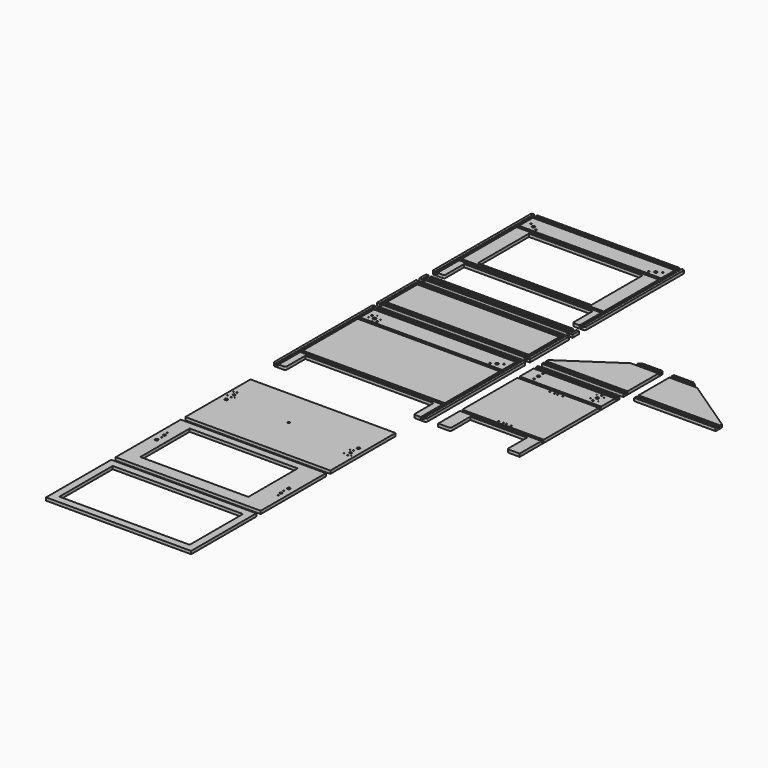
from build123d import *

# Parameters (mm, degrees)
F0_W     = 576
F0_H     = 12
F0_W_2   = 10
F0_H_2   = 505
F0_H_3   = 70
F0_W_3   = 460
F0_H_4   = 50
F0_H_5   = 10
F0_H_6   = 279
F0_H_7   = 259
F0_W_4   = 6
F1_DEPTH = 12
F0_W_5   = 330
F0_W_6   = 588
F0_H_8   = 330
F0_R     = 4.7874665738
F0_W_7   = 438
F0_H_9   = 250
F0_W_8   = 528
F0_H_10  = 270
F0_H_11  = 156
F0_W_9   = 12
F2_DEPTH = 6
F3_R     = 6
F3_R_2   = 2.5
F3_R_3   = 3.3
F3_R_4   = 5
F4_DEPTH = 25
F5_R     = 7
F5_2_R   = 7
F5_3_R   = 7
F6_R     = 1.5
F7_DEPTH = 25


with BuildPart() as f1:
    # F0 (on Top) → F1 (new body)
    with BuildSketch(Plane.XY):
        with Locations((151.8414666056, 1212)):
            Rectangle(F0_W, F0_H)
        with Locations((456.8414666056, 1057.5)):
            Rectangle(F0_W_2, F0_H_2)
        with Locations((151.8414666056, 921)):
            Rectangle(F0_W, F0_H)
        with Locations((151.8414666056, 1253)):
            Rectangle(F0_W, F0_H_3)
        with Locations((151.8414666056, 1253)):
            Rectangle(F0_W_3, F0_H_4, mode=Mode.SUBTRACT)
        with Locations((151.8414666056, 1305)):
            Rectangle(F0_W, F0_H_5)
        with Locations((151.8414666056, 1294)):
            Rectangle(F0_W, F0_H)
        with Locations((151.8414666056, 1066.5)):
            Rectangle(F0_W, F0_H_6)
        with Locations((151.8414666056, 1066.5)):
            Rectangle(F0_W_3, F0_H_7, mode=Mode.SUBTRACT)
        Polygon((-136.1585333944, 915), (-136.1585333944, 805), (-108.1585333944, 805), (-108.1585333944, 905), (411.8414666056, 905), (411.8414666056, 805), (439.8414666056, 805), (439.8414666056, 915), align=None)
        with Locations((-153.1585333944, 1057.5)):
            Rectangle(F0_W_2, F0_H_2)
        Polygon((-148.1585333944, 1310), (-148.1585333944, 805), (-136.1585333944, 805), (-136.1585333944, 915), (-142.1585333944, 915), (-142.1585333944, 927), (-136.1585333944, 927), (-136.1585333944, 1206), (-142.1585333944, 1206), (-142.1585333944, 1218), (-136.1585333944, 1218), (-136.1585333944, 1288), (-142.1585333944, 1288), (-142.1585333944, 1300), (-136.1585333944, 1300), (-136.1585333944, 1310), align=None)
        Polygon((451.8414666056, 1310), (439.8414666056, 1310), (439.8414666056, 1300), (445.8414666056, 1300), (445.8414666056, 1288), (439.8414666056, 1288), (439.8414666056, 1218), (445.8414666056, 1218), (445.8414666056, 1206), (439.8414666056, 1206), (439.8414666056, 927), (445.8414666056, 927), (445.8414666056, 915), (439.8414666056, 915), (439.8414666056, 805), (451.8414666056, 805), align=None)
        with Locations((442.8414666056, 921)):
            Rectangle(F0_W_4, F0_H)
        with Locations((-139.1585333944, 1212)):
            Rectangle(F0_W_4, F0_H)
        with Locations((442.8414666056, 1294)):
            Rectangle(F0_W_4, F0_H)
        with Locations((442.8414666056, 1212)):
            Rectangle(F0_W_4, F0_H)
        with Locations((-139.1585333944, 1294)):
            Rectangle(F0_W_4, F0_H)
        with Locations((-139.1585333944, 921)):
            Rectangle(F0_W_4, F0_H)
        with Locations((151.8414666056, 1253)):
            Rectangle(F0_W_3, F0_H_4)
    extrude(amount=-F1_DEPTH)


with BuildPart() as f1b:
    # F0 (on Top) → F1, piece 2 (new body)
    with BuildSketch(Plane.XY):
        with Locations((675.8917057514, 448)):
            Rectangle(F0_W_5, F0_H_3)
        with Locations((675.8917057514, 261.5)):
            Rectangle(F0_W_5, F0_H_6)
        with Locations((675.8917057514, 407)):
            Rectangle(F0_W_5, F0_H)
        Polygon((510.8917057514, 110), (510.8917057514, 0), (560.8917057514, 0), (560.8917057514, 100), (790.8917057514, 100), (790.8917057514, 0), (840.8917057514, 0), (840.8917057514, 110), align=None)
        with Locations((675.8917057514, 116)):
            Rectangle(F0_W_5, F0_H)
        with Locations((675.8917057514, 500)):
            Rectangle(F0_W_5, F0_H_5)
        with Locations((675.8917057514, 489)):
            Rectangle(F0_W_5, F0_H)
    extrude(amount=-F1_DEPTH)


with BuildPart() as f1c:
    # F0 (on Top) → F1, piece 3 (new body)
    with BuildSketch(Plane.XY):
        with Locations((151.8414666056, 261.5)):
            Rectangle(F0_W, F0_H_6)
        with Locations((151.8414666056, 500)):
            Rectangle(F0_W, F0_H_5)
        Polygon((-136.1585333944, 110), (-136.1585333944, 0), (-108.1585333944, 0), (-108.1585333944, 100), (411.8414666056, 100), (411.8414666056, 0), (439.8414666056, 0), (439.8414666056, 110), align=None)
        with Locations((151.8414666056, 407)):
            Rectangle(F0_W, F0_H)
        with Locations((151.8414666056, 448)):
            Rectangle(F0_W, F0_H_3)
        with Locations((-153.1585333944, 252.5)):
            Rectangle(F0_W_2, F0_H_2)
        with Locations((151.8414666056, 489)):
            Rectangle(F0_W, F0_H)
        with Locations((151.8414666056, 116)):
            Rectangle(F0_W, F0_H)
        with Locations((-139.1585333944, 407)):
            Rectangle(F0_W_4, F0_H)
        with Locations((-139.1585333944, 116)):
            Rectangle(F0_W_4, F0_H)
        with Locations((-139.1585333944, 489)):
            Rectangle(F0_W_4, F0_H)
        with Locations((456.8414666056, 252.5)):
            Rectangle(F0_W_2, F0_H_2)
        with Locations((442.8414666056, 489)):
            Rectangle(F0_W_4, F0_H)
        with Locations((442.8414666056, 116)):
            Rectangle(F0_W_4, F0_H)
        with Locations((442.8414666056, 407)):
            Rectangle(F0_W_4, F0_H)
        Polygon((-148.1585333944, 505), (-148.1585333944, 0), (-136.1585333944, 0), (-136.1585333944, 110), (-142.1585333944, 110), (-142.1585333944, 122), (-136.1585333944, 122), (-136.1585333944, 401), (-142.1585333944, 401), (-142.1585333944, 413), (-136.1585333944, 413), (-136.1585333944, 483), (-142.1585333944, 483), (-142.1585333944, 495), (-136.1585333944, 495), (-136.1585333944, 505), align=None)
        Polygon((451.8414666056, 505), (439.8414666056, 505), (439.8414666056, 495), (445.8414666056, 495), (445.8414666056, 483), (439.8414666056, 483), (439.8414666056, 413), (445.8414666056, 413), (445.8414666056, 401), (439.8414666056, 401), (439.8414666056, 122), (445.8414666056, 122), (445.8414666056, 110), (439.8414666056, 110), (439.8414666056, 0), (451.8414666056, 0), align=None)
    extrude(amount=-F1_DEPTH)


with BuildPart() as f1d:
    # F0 (on Top) → F1, piece 4 (new body)
    with BuildSketch(Plane.XY):
        with Locations((151.8414666056, -300.2730111413)):
            Rectangle(F0_W_6, F0_H_8)
        with Locations((136.8414666056, -290.2730111413)):
            Circle(F0_R, mode=Mode.SUBTRACT)
    extrude(amount=-F1_DEPTH)


with BuildPart() as f1e:
    # F0 (on Top) → F1, piece 5 (new body)
    with BuildSketch(Plane.XY):
        with Locations((151.8414666056, -653.3492064476)):
            Rectangle(F0_W_6, F0_H_8)
        with Locations((136.8414666056, -643.3492064476)):
            Rectangle(F0_W_7, F0_H_9, mode=Mode.SUBTRACT)
    extrude(amount=-F1_DEPTH)


with BuildPart() as f1f:
    # F0 (on Top) → F1, piece 6 (new body)
    with BuildSketch(Plane.XY):
        with Locations((151.8414666056, -1005.8201861382)):
            Rectangle(F0_W_6, F0_H_8)
        with Locations((151.8414666056, -1005.8201861382)):
            Rectangle(F0_W_8, F0_H_10, mode=Mode.SUBTRACT)
    extrude(amount=-F1_DEPTH)


with BuildPart() as f1g:
    # F0 (on Top) → F1, piece 7 (new body)
    with BuildSketch(Plane.XY):
        Polygon((510.8917057514, 557), (510.8917057514, 547), (840.8917057514, 547), (840.8917057514, 703), (728.1536105133, 703), align=None)
        Polygon((728.1536105133, 703), (840.8917057514, 703), (840.8917057514, 715), (746.0107533705, 715), align=None)
        Polygon((746.0107533705, 715), (840.8917057514, 715), (840.8917057514, 725), (760.8917057514, 725), align=None)
        with Locations((675.8917057514, 530)):
            Rectangle(F0_W_5, F0_H_5)
        with Locations((675.8917057514, 541)):
            Rectangle(F0_W_5, F0_H)
    extrude(amount=-F1_DEPTH)


with BuildPart() as f1h:
    # F0 (on Top) → F1, piece 8 (new body)
    with BuildSketch(Plane.XY):
        Polygon((885.1829600334, 703), (885.1829600334, 547), (1215.1829600334, 547), (1215.1829600334, 557), (997.9210552715, 703), align=None)
        Polygon((885.1829600334, 725), (885.1829600334, 715), (980.0639124144, 715), (965.1829600334, 725), align=None)
        Polygon((885.1829600334, 715), (885.1829600334, 703), (997.9210552715, 703), (980.0639124144, 715), align=None)
        with Locations((1050.1829600334, 530)):
            Rectangle(F0_W_5, F0_H_5)
        with Locations((1050.1829600334, 541)):
            Rectangle(F0_W_5, F0_H)
    extrude(amount=-F1_DEPTH)


with BuildPart() as f1i:
    # F0 (on Top) → F1, piece 9 (new body)
    with BuildSketch(Plane.XY):
        with Locations((151.8414666056, 625)):
            Rectangle(F0_W, F0_H_11)
        with Locations((151.8414666056, 709)):
            Rectangle(F0_W, F0_H)
        with Locations((151.8414666056, 720)):
            Rectangle(F0_W, F0_H_5)
        with Locations((-142.1585333944, 720)):
            Rectangle(F0_W_9, F0_H_5)
        with Locations((-142.1585333944, 709)):
            Rectangle(F0_W_9, F0_H)
        with Locations((-142.1585333944, 625)):
            Rectangle(F0_W_9, F0_H_11)
        Polygon((-148.1585333944, 725), (-158.1585333944, 725), (-158.1585333944, 525), (-148.1585333944, 525), (-148.1585333944, 535), (-148.1585333944, 547), (-148.1585333944, 703), (-148.1585333944, 715), align=None)
        Polygon((461.8414666056, 725), (451.8414666056, 725), (451.8414666056, 715), (451.8414666056, 703), (451.8414666056, 547), (451.8414666056, 535), (451.8414666056, 525), (461.8414666056, 525), align=None)
        with Locations((445.8414666056, 720)):
            Rectangle(F0_W_9, F0_H_5)
        with Locations((445.8414666056, 709)):
            Rectangle(F0_W_9, F0_H)
        with Locations((445.8414666056, 625)):
            Rectangle(F0_W_9, F0_H_11)
        with Locations((151.8414666056, 530)):
            Rectangle(F0_W, F0_H_5)
        with Locations((151.8414666056, 541)):
            Rectangle(F0_W, F0_H)
        with Locations((445.8414666056, 541)):
            Rectangle(F0_W_9, F0_H)
        with Locations((445.8414666056, 530)):
            Rectangle(F0_W_9, F0_H_5)
        with Locations((-142.1585333944, 541)):
            Rectangle(F0_W_9, F0_H)
        with Locations((-142.1585333944, 530)):
            Rectangle(F0_W_9, F0_H_5)
    extrude(amount=-F1_DEPTH)


with BuildPart() as f1j:
    # F0 (on Top) → F1, piece 10 (new body)
    with BuildSketch(Plane.XY):
        with Locations((151.8414666056, 768.795539856)):
            Rectangle(F0_W, F0_H_5)
        with Locations((151.8414666056, 757.795539856)):
            Rectangle(F0_W, F0_H)
        with Locations((151.8414666056, 746.795539856)):
            Rectangle(F0_W, F0_H_5)
        with Locations((445.8414666056, 757.795539856)):
            Rectangle(F0_W_9, F0_H)
        Polygon((451.8414666056, 751.795539856), (451.8414666056, 741.795539856), (461.8414666056, 741.795539856), (461.8414666056, 773.795539856), (451.8414666056, 773.795539856), (451.8414666056, 763.795539856), align=None)
        with Locations((445.8414666056, 746.795539856)):
            Rectangle(F0_W_9, F0_H_5)
        with Locations((445.8414666056, 768.795539856)):
            Rectangle(F0_W_9, F0_H_5)
        Polygon((-158.1585333944, 773.795539856), (-158.1585333944, 741.795539856), (-148.1585333944, 741.795539856), (-148.1585333944, 751.795539856), (-148.1585333944, 763.795539856), (-148.1585333944, 773.795539856), align=None)
        with Locations((-142.1585333944, 757.795539856)):
            Rectangle(F0_W_9, F0_H)
        with Locations((-142.1585333944, 768.795539856)):
            Rectangle(F0_W_9, F0_H_5)
        with Locations((-142.1585333944, 746.795539856)):
            Rectangle(F0_W_9, F0_H_5)
    extrude(amount=-F1_DEPTH)


with BuildPart() as f2_tool:
    # F0 (on Top) → F2 (new body)
    with BuildSketch(Plane.XY):
        with Locations((151.8414666056, 1212)):
            Rectangle(F0_W, F0_H)
        with Locations((151.8414666056, 1294)):
            Rectangle(F0_W, F0_H)
        with Locations((151.8414666056, 921)):
            Rectangle(F0_W, F0_H)
        Polygon((-148.1585333944, 1310), (-148.1585333944, 805), (-136.1585333944, 805), (-136.1585333944, 915), (-142.1585333944, 915), (-142.1585333944, 927), (-136.1585333944, 927), (-136.1585333944, 1206), (-142.1585333944, 1206), (-142.1585333944, 1218), (-136.1585333944, 1218), (-136.1585333944, 1288), (-142.1585333944, 1288), (-142.1585333944, 1300), (-136.1585333944, 1300), (-136.1585333944, 1310), align=None)
        with Locations((-139.1585333944, 921)):
            Rectangle(F0_W_4, F0_H)
        with Locations((-139.1585333944, 1212)):
            Rectangle(F0_W_4, F0_H)
        with Locations((-139.1585333944, 1294)):
            Rectangle(F0_W_4, F0_H)
        with Locations((442.8414666056, 1294)):
            Rectangle(F0_W_4, F0_H)
        with Locations((442.8414666056, 1212)):
            Rectangle(F0_W_4, F0_H)
        Polygon((451.8414666056, 1310), (439.8414666056, 1310), (439.8414666056, 1300), (445.8414666056, 1300), (445.8414666056, 1288), (439.8414666056, 1288), (439.8414666056, 1218), (445.8414666056, 1218), (445.8414666056, 1206), (439.8414666056, 1206), (439.8414666056, 927), (445.8414666056, 927), (445.8414666056, 915), (439.8414666056, 915), (439.8414666056, 805), (451.8414666056, 805), align=None)
        with Locations((442.8414666056, 921)):
            Rectangle(F0_W_4, F0_H)
        with Locations((151.8414666056, 757.795539856)):
            Rectangle(F0_W, F0_H)
        with Locations((-142.1585333944, 757.795539856)):
            Rectangle(F0_W_9, F0_H)
        with Locations((-142.1585333944, 768.795539856)):
            Rectangle(F0_W_9, F0_H_5)
        with Locations((-142.1585333944, 746.795539856)):
            Rectangle(F0_W_9, F0_H_5)
        with Locations((445.8414666056, 768.795539856)):
            Rectangle(F0_W_9, F0_H_5)
        with Locations((445.8414666056, 757.795539856)):
            Rectangle(F0_W_9, F0_H)
        with Locations((445.8414666056, 746.795539856)):
            Rectangle(F0_W_9, F0_H_5)
        with Locations((151.8414666056, 709)):
            Rectangle(F0_W, F0_H)
        with Locations((151.8414666056, 541)):
            Rectangle(F0_W, F0_H)
        with Locations((-142.1585333944, 625)):
            Rectangle(F0_W_9, F0_H_11)
        with Locations((445.8414666056, 625)):
            Rectangle(F0_W_9, F0_H_11)
        with Locations((445.8414666056, 720)):
            Rectangle(F0_W_9, F0_H_5)
        with Locations((445.8414666056, 709)):
            Rectangle(F0_W_9, F0_H)
        with Locations((445.8414666056, 541)):
            Rectangle(F0_W_9, F0_H)
        with Locations((445.8414666056, 530)):
            Rectangle(F0_W_9, F0_H_5)
        with Locations((-142.1585333944, 530)):
            Rectangle(F0_W_9, F0_H_5)
        with Locations((-142.1585333944, 541)):
            Rectangle(F0_W_9, F0_H)
        with Locations((-142.1585333944, 709)):
            Rectangle(F0_W_9, F0_H)
        with Locations((-142.1585333944, 720)):
            Rectangle(F0_W_9, F0_H_5)
        with Locations((151.8414666056, 489)):
            Rectangle(F0_W, F0_H)
        with Locations((151.8414666056, 407)):
            Rectangle(F0_W, F0_H)
        with Locations((151.8414666056, 116)):
            Rectangle(F0_W, F0_H)
        Polygon((-148.1585333944, 505), (-148.1585333944, 0), (-136.1585333944, 0), (-136.1585333944, 110), (-142.1585333944, 110), (-142.1585333944, 122), (-136.1585333944, 122), (-136.1585333944, 401), (-142.1585333944, 401), (-142.1585333944, 413), (-136.1585333944, 413), (-136.1585333944, 483), (-142.1585333944, 483), (-142.1585333944, 495), (-136.1585333944, 495), (-136.1585333944, 505), align=None)
        Polygon((451.8414666056, 505), (439.8414666056, 505), (439.8414666056, 495), (445.8414666056, 495), (445.8414666056, 483), (439.8414666056, 483), (439.8414666056, 413), (445.8414666056, 413), (445.8414666056, 401), (439.8414666056, 401), (439.8414666056, 122), (445.8414666056, 122), (445.8414666056, 110), (439.8414666056, 110), (439.8414666056, 0), (451.8414666056, 0), align=None)
        with Locations((-139.1585333944, 489)):
            Rectangle(F0_W_4, F0_H)
        with Locations((-139.1585333944, 407)):
            Rectangle(F0_W_4, F0_H)
        with Locations((-139.1585333944, 116)):
            Rectangle(F0_W_4, F0_H)
        with Locations((442.8414666056, 489)):
            Rectangle(F0_W_4, F0_H)
        with Locations((442.8414666056, 407)):
            Rectangle(F0_W_4, F0_H)
        with Locations((442.8414666056, 116)):
            Rectangle(F0_W_4, F0_H)
        Polygon((728.1536105133, 703), (840.8917057514, 703), (840.8917057514, 715), (746.0107533705, 715), align=None)
        Polygon((885.1829600334, 715), (885.1829600334, 703), (997.9210552715, 703), (980.0639124144, 715), align=None)
        with Locations((1050.1829600334, 541)):
            Rectangle(F0_W_5, F0_H)
        with Locations((675.8917057514, 541)):
            Rectangle(F0_W_5, F0_H)
        with Locations((675.8917057514, 489)):
            Rectangle(F0_W_5, F0_H)
        with Locations((675.8917057514, 407)):
            Rectangle(F0_W_5, F0_H)
        with Locations((675.8917057514, 116)):
            Rectangle(F0_W_5, F0_H)
    extrude(amount=-F2_DEPTH)


with BuildPart() as f1_1:
    add(f1.part)

    # F2: cut by f2_tool
    add(f2_tool.part, mode=Mode.SUBTRACT)


with BuildPart() as f1b_1:
    add(f1b.part)

    # F2: cut by f2_tool
    add(f2_tool.part, mode=Mode.SUBTRACT)


with BuildPart() as f1c_1:
    add(f1c.part)

    # F2: cut by f2_tool
    add(f2_tool.part, mode=Mode.SUBTRACT)


with BuildPart() as f1g_1:
    add(f1g.part)

    # F2: cut by f2_tool
    add(f2_tool.part, mode=Mode.SUBTRACT)


with BuildPart() as f1h_1:
    add(f1h.part)

    # F2: cut by f2_tool
    add(f2_tool.part, mode=Mode.SUBTRACT)


with BuildPart() as f1i_1:
    add(f1i.part)

    # F2: cut by f2_tool
    add(f2_tool.part, mode=Mode.SUBTRACT)


with BuildPart() as f1j_1:
    add(f1j.part)

    # F2: cut by f2_tool
    add(f2_tool.part, mode=Mode.SUBTRACT)


with BuildPart() as f4_tool:
    # F3 (on face) → F4 (new body)
    with BuildSketch(Plane.XY):
        with Locations((-96.1585333944, 1241)):
            Circle(F3_R)
        with Locations((399.8414666056, 1241)):
            Circle(F3_R)
        with Locations((-96.1585333944, 436)):
            Circle(F3_R)
        with Locations((399.8414666056, 436)):
            Circle(F3_R)
        with Locations((556.8917057514, 451)):
            Circle(F3_R)
        with Locations((794.8917057514, 451)):
            Circle(F3_R)
        with Locations((48.5081332723, 489)):
            Circle(F3_R_2)
        with Locations((255.174799939, 489)):
            Circle(F3_R_2)
        with Locations((48.5081332723, 407)):
            Circle(F3_R_2)
        with Locations((255.174799939, 407)):
            Circle(F3_R_2)
        with Locations((48.5081332723, 116)):
            Circle(F3_R_2)
        with Locations((255.174799939, 116)):
            Circle(F3_R_2)
        with Locations((620.8917057514, 489)):
            Circle(F3_R_2)
        with Locations((730.8917057514, 489)):
            Circle(F3_R_2)
        with Locations((620.8917057514, 407)):
            Circle(F3_R_2)
        with Locations((730.8917057514, 407)):
            Circle(F3_R_2)
        with Locations((620.8917057514, 116)):
            Circle(F3_R_2)
        with Locations((730.8917057514, 116)):
            Circle(F3_R_2)
        with Locations((-142.1585333944, 50)):
            Circle(F3_R_2)
        with Locations((445.8414666056, 50)):
            Circle(F3_R_2)
        with Locations((-142.1585333944, 855)):
            Circle(F3_R_2)
        with Locations((445.8414666056, 855)):
            Circle(F3_R_2)
        with Locations((48.5081332723, 1212)):
            Circle(F3_R_2)
        with Locations((255.174799939, 1212)):
            Circle(F3_R_2)
        with Locations((48.5081332723, 921)):
            Circle(F3_R_2)
        with Locations((255.174799939, 921)):
            Circle(F3_R_2)
        with Locations((255.174799939, 1294)):
            Circle(F3_R_2)
        with Locations((48.5081332723, 1294)):
            Circle(F3_R_2)
        with Locations((-142.1585333944, 261.5)):
            Circle(F3_R_2)
        with Locations((445.8414666056, 261.5)):
            Circle(F3_R_2)
        with Locations((-142.1585333944, 448)):
            Circle(F3_R_2)
        with Locations((445.8414666056, 448)):
            Circle(F3_R_2)
        with Locations((-142.1585333944, 1253)):
            Circle(F3_R_2)
        with Locations((445.8414666056, 1253)):
            Circle(F3_R_2)
        with Locations((445.8414666056, 1066.5)):
            Circle(F3_R_2)
        with Locations((-142.1585333944, 1066.5)):
            Circle(F3_R_2)
        with Locations((-115.6441049795, 447.25)):
            Circle(F3_R_3)
        with Locations((-115.6441049795, 1252.25)):
            Circle(F3_R_3)
        with Locations((-76.6729618092, 1229.75)):
            Circle(F3_R_3)
        with Locations((380.3558950205, 1229.75)):
            Circle(F3_R_3)
        with Locations((419.3270381908, 1252.25)):
            Circle(F3_R_3)
        with Locations((380.3558950205, 424.75)):
            Circle(F3_R_3)
        with Locations((419.3270381908, 447.25)):
            Circle(F3_R_3)
        with Locations((-76.6729618092, 424.75)):
            Circle(F3_R_3)
        with Locations((556.8917057514, 473.5)):
            Circle(F3_R_3)
        with Locations((556.8917057514, 428.5)):
            Circle(F3_R_3)
        with Locations((794.8917057514, 428.5)):
            Circle(F3_R_3)
        with Locations((794.8917057514, 473.5)):
            Circle(F3_R_3)
        with Locations((669.8917057514, 391)):
            Circle(F3_R_2)
        with Locations((681.8917057514, 391)):
            Circle(F3_R_2)
        with Locations((681.8917057514, 132)):
            Circle(F3_R_2)
        with Locations((669.8917057514, 132)):
            Circle(F3_R_2)
        with Locations((701.8917057514, 391)):
            Circle(F3_R_2)
        with Locations((649.8917057514, 391)):
            Circle(F3_R_2)
        with Locations((701.8917057514, 132)):
            Circle(F3_R_2)
        with Locations((649.8917057514, 132)):
            Circle(F3_R_2)
        with Locations((-119.3276126368, -232.3002696488)):
            Circle(F3_R_2)
        with Locations((-112.9894541519, -268.2457526338)):
            Circle(F3_R_2)
        with Locations((-116.1585333944, -250.2730111413)):
            Circle(F3_R_4)
        with Locations((416.6723873632, -312.3002696488)):
            Circle(F3_R_2)
        with Locations((419.8414666056, -330.2730111413)):
            Circle(F3_R_4)
        with Locations((423.0105458481, -348.2457526338)):
            Circle(F3_R_2)
        with Locations((423.0105458481, -701.3219479401)):
            Circle(F3_R_2)
        with Locations((416.6723873632, -665.3764649551)):
            Circle(F3_R_2)
        with Locations((419.8414666056, -683.3492064476)):
            Circle(F3_R_4)
        with Locations((-116.1585333944, -603.3492064476)):
            Circle(F3_R_4)
        with Locations((-112.9894541519, -621.3219479401)):
            Circle(F3_R_2)
        with Locations((-119.3276126368, -585.3764649551)):
            Circle(F3_R_2)
        with Locations((419.8414666056, -290.2730111413)):
            Circle(F3_R)
        with Locations((-116.1585333944, -290.2730111413)):
            Circle(F3_R)
        with Locations((-116.1585333944, -643.3492064476)):
            Circle(F3_R)
        with Locations((419.8414666056, -643.3492064476)):
            Circle(F3_R)
    extrude(amount=-F4_DEPTH)


with BuildPart() as f1_2:
    add(f1_1.part)

    # F4: cut by f4_tool
    add(f4_tool.part, mode=Mode.SUBTRACT)

    # F5
    f5_edges = [f1_2.edges().sort_by_distance(p)[0] for p in [
        (461.841467, 1310, -6),
        (-158.158533, 1310, -6),
        (-158.158533, 805, -6),
        (-108.158533, 805, -6),
        (461.841467, 805, -6),
        (411.841467, 805, -6),
    ]]
    fillet(f5_edges, radius=F5_R)


with BuildPart() as f1b_2:
    add(f1b_1.part)

    # F4: cut by f4_tool
    add(f4_tool.part, mode=Mode.SUBTRACT)

    # F5#2
    f5_2_edges = [f1b_2.edges().sort_by_distance(p)[0] for p in [
        (560.891706, 0, -6),
        (790.891706, 0, -6),
    ]]
    fillet(f5_2_edges, radius=F5_2_R)


with BuildPart() as f1c_2:
    add(f1c_1.part)

    # F4: cut by f4_tool
    add(f4_tool.part, mode=Mode.SUBTRACT)

    # F5#3
    f5_3_edges = [f1c_2.edges().sort_by_distance(p)[0] for p in [
        (411.841467, 0, -6),
        (-108.158533, 0, -6),
        (-158.158533, 0, -6),
        (461.841467, 0, -6),
        (-158.158533, 505, -6),
        (461.841467, 505, -6),
    ]]
    fillet(f5_3_edges, radius=F5_3_R)


with BuildPart() as f1d_1:
    add(f1d.part)

    # F4: cut by f4_tool
    add(f4_tool.part, mode=Mode.SUBTRACT)


with BuildPart() as f1e_1:
    add(f1e.part)

    # F4: cut by f4_tool
    add(f4_tool.part, mode=Mode.SUBTRACT)


with BuildPart() as f7_tool:
    # F6 (on Top) → F7 (new body)
    with BuildSketch(Plane.XY):
        with Locations((-116.6489144511, 430.5096189432)):
            Circle(F6_R)
        with Locations((-101.6489144511, 456.4903810568)):
            Circle(F6_R)
        with Locations((-90.6681523376, 415.5096189432)):
            Circle(F6_R)
        with Locations((-75.6681523376, 441.4903810568)):
            Circle(F6_R)
        with Locations((779.8917057514, 466)):
            Circle(F6_R)
        with Locations((779.8917057514, 436)):
            Circle(F6_R)
        with Locations((809.8917057514, 436)):
            Circle(F6_R)
        with Locations((809.8917057514, 466)):
            Circle(F6_R)
        with Locations((-101.1585333944, -265.2730111413)):
            Circle(F6_R)
        with Locations((-131.1585333944, -265.2730111413)):
            Circle(F6_R)
        with Locations((-131.1585333944, -235.2730111413)):
            Circle(F6_R)
        with Locations((-101.1585333944, -235.2730111413)):
            Circle(F6_R)
        with Locations((404.8414666056, -315.2730111413)):
            Circle(F6_R)
        with Locations((434.8414666056, -315.2730111413)):
            Circle(F6_R)
        with Locations((434.8414666056, -345.2730111413)):
            Circle(F6_R)
        with Locations((404.8414666056, -345.2730111413)):
            Circle(F6_R)
    extrude(amount=-F7_DEPTH)


with BuildPart() as f1b_3:
    add(f1b_2.part)

    # F7: cut by f7_tool
    add(f7_tool.part, mode=Mode.SUBTRACT)


with BuildPart() as f1c_3:
    add(f1c_2.part)

    # F7: cut by f7_tool
    add(f7_tool.part, mode=Mode.SUBTRACT)


with BuildPart() as f1d_2:
    add(f1d_1.part)

    # F7: cut by f7_tool
    add(f7_tool.part, mode=Mode.SUBTRACT)


solid = Compound([f1f.part, f1g_1.part, f1h_1.part, f1i_1.part, f1j_1.part, f1_2.part, f1e_1.part, f1b_3.part, f1c_3.part, f1d_2.part])
